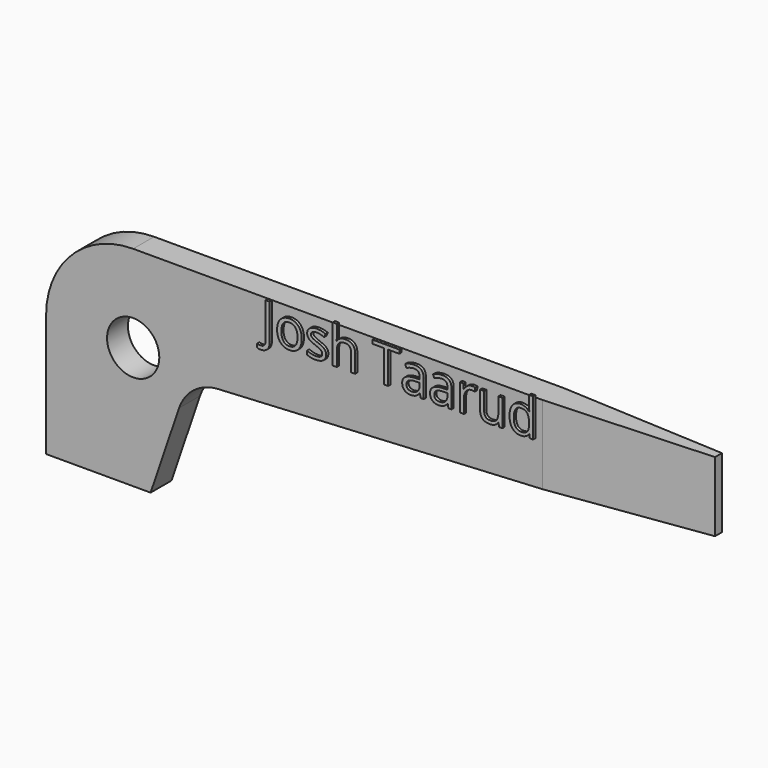
from build123d import *

# Parameters (mm, degrees)
F1_DEPTH     = 2.38125
F2_R         = 2.38125
F3_DEPTH     = 2.38225
F5_DEPTH     = 25.4
F6_TEXT_SIZE = 4.563141815
F7_DEPTH     = 0.254


# Not quite as in the source:
# - Text() gives the source's letters only with a copy of the font that has no kerning and outlines rounded to 1/6400 em; it was checked with that copy


with BuildPart() as f1:
    # F0 (on Front) → F1 (new body)
    with BuildSketch(Plane.XZ):
        with BuildLine():
            Line((60.325, 19.05), (7.9375, 19.05))
            ThreePointArc((7.9375, 19.05), (2.3248399243, 16.7251600757), (0, 11.1125))
            Line((0, 11.1125), (0, 0))
            Line((0, 0), (9.525, 0))
            Line((9.525, 0), (12.1173647876, 7.6271664624))
            ThreePointArc((12.1173647876, 7.6271664624), (13.4786145605, 9.5135918491), (15.6631963617, 10.3130942181))
            Line((15.6631963617, 10.3130942181), (60.325, 12.7))
            Line((60.325, 12.7), (60.325, 19.05))
        make_face()
    extrude(amount=F1_DEPTH)

    # F2 (on face) → F3 (cut, through all)
    with BuildSketch(Plane.XZ.offset(2.38125)):
        with Locations((7.9375, 11.1125)):
            Circle(F2_R)
    extrude(amount=-F3_DEPTH, mode=Mode.SUBTRACT)

    # F4 (on face) → F5 (cut)
    with BuildSketch(Plane.XY.offset(19.05)):
        Polygon((60.325, -0.79375), (60.325, 0), (45.24375, 0), align=None)
        Polygon((60.325, -2.38125), (60.325, -1.5875), (45.24375, -2.38125), align=None)
    extrude(amount=-F5_DEPTH, mode=Mode.SUBTRACT)

    # F6 (on face) → F7 (join)
    with BuildSketch(Plane.XZ.offset(2.38125)):
        with Locations((19.7856966179, 15.7645378932)):
            Text('Josh Taarud', F6_TEXT_SIZE, font='Open Sans', text_align=(TextAlign.LEFT, TextAlign.BOTTOM))
    extrude(amount=F7_DEPTH)


solid = f1.part
